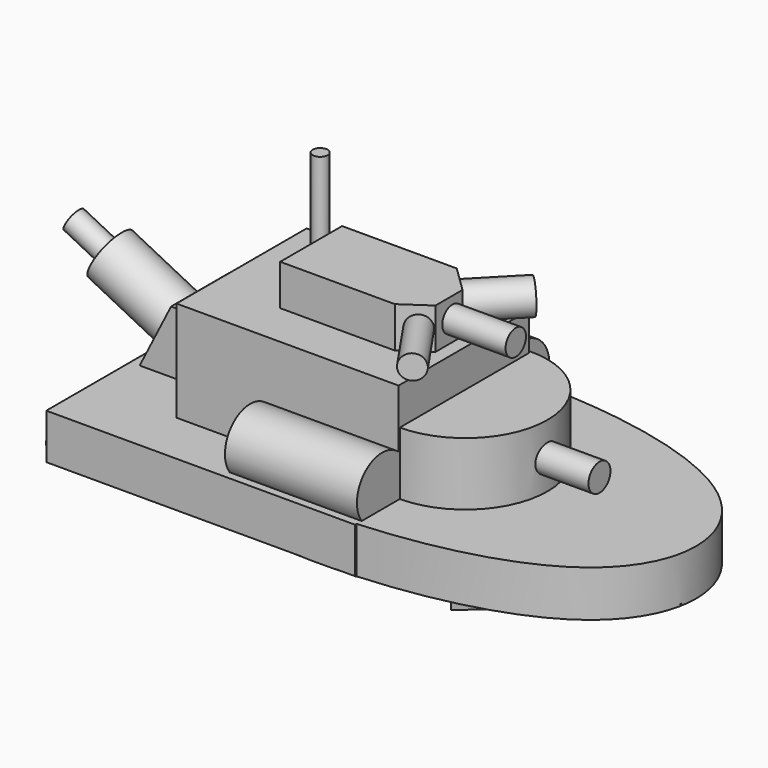
from build123d import *

# Parameters (mm, degrees)
F0_W      = 281.3238278031
F0_H      = 100.6183102727
F1_DEPTH  = 28.702
F3_DEPTH  = 192.024
F5_DEPTH  = 11.176
F6_DEPTH  = 16.51
F7_R      = 50.9790191052
F8_DEPTH  = 39.116
F9_W      = 138.0599290133
F9_H      = 101.1783219874
F10_DEPTH = 62.484
F11_R     = 8.5441952261
F12_DEPTH = 83.312
F13_W     = 61.6130270064
F13_H     = 25.6704241037
F14_DEPTH = 29.464
F15_W     = 38.1111055613
F15_H     = 22.8097289801
F16_DEPTH = 25.4
F17_R     = 21.1546629921
F18_DEPTH = 63.246
F19_R     = 19.5556802918
F20_DEPTH = 82.042
F21_W     = 71.2716747075
F21_H     = 48.0869095773
F22_DEPTH = 25.4
F23_R     = 7.9233421665
F24_DEPTH = 39.37
F25_R     = 7.5156557612
F26_DEPTH = 40.894
F27_R     = 10.3119477228
F28_DEPTH = 36.322
F29_W     = 44.719548896
F29_H     = 38.6362597346
F30_DEPTH = 28.702
F32_DEPTH = 44.958
F33_R     = 15.6273286388
F34_DEPTH = 49.53
F35_R     = 7.0493899226
F36_DEPTH = 25.4
F37_R     = 13.7507594289
F37_R_2   = 7.9743442037
F38_DEPTH = 37.592
F37_R_3   = 8.7506805575
F39_R     = 4.644151777
F40_DEPTH = 58.166


with BuildPart() as f1:
    # F0 (on Top) → F1 (new body)
    with BuildSketch(Plane.XY):
        with Locations((-24.3793539703, 0.1091174781)):
            Rectangle(F0_W, F0_H)
        with BuildLine():
            add(Edge.make_bspline(
                [(116.2825599313, 50.4182726145), (152.293026111, 22.4535704341), (152.293026111, -22.2353354778), (116.2825599313, -50.2000376582)],
                knots=[0.3128819291, 0.3128819291, 0.3128819291, 0.3128819291, 0.5, 0.5, 0.5, 0.5], degree=3))
            Line((116.2825599313, 50.4182726145), (116.2825599313, -50.2000376582))
        make_face()
        with BuildLine():
            Line((-165.0412678719, 50.4182726145), (116.2825599313, 50.4182726145))
            add(Edge.make_bspline(
                [(-165.0412678719, 50.4182726145), (-104.8278204483, 97.1783205419), (56.0691125078, 97.1783205419), (116.2825599313, 50.4182726145)],
                knots=[0, 0, 0, 0, 0.3128819291, 0.3128819291, 0.3128819291, 0.3128819291], degree=3))
        make_face()
        with BuildLine():
            Line((-165.0412678719, -50.2000376582), (-165.0412678719, 50.4182726145))
            add(Edge.make_bspline(
                [(-165.0412678719, -50.2000376582), (-201.0517340516, -22.2353354778), (-201.0517340516, 22.4535704341), (-165.0412678719, 50.4182726145)],
                knots=[0.8128819291, 0.8128819291, 0.8128819291, 0.8128819291, 1, 1, 1, 1], degree=3))
        make_face()
        with BuildLine():
            add(Edge.make_bspline(
                [(116.2825599313, -50.2000376582), (56.0691125078, -96.9600855856), (-104.8278204483, -96.9600855856), (-165.0412678719, -50.2000376582)],
                knots=[0.5, 0.5, 0.5, 0.5, 0.8128819291, 0.8128819291, 0.8128819291, 0.8128819291], degree=3))
            Line((116.2825599313, -50.2000376582), (-165.0412678719, -50.2000376582))
        make_face()
    extrude(amount=-F1_DEPTH)

    # F2 (on Right) → F3 (join)
    with BuildSketch(Plane.YZ):
        Polygon((84.8256722093, -28.180513531), (84.8256722093, 0), (-85.6735184789, 0), (-85.6735184789, -28.180513531), (0, -75.7616832852), align=None)
    extrude(amount=-F3_DEPTH)

    # F4 (on Front) → F5 (join)
    with BuildSketch(Plane.XZ):
        Polygon((0, -27.5897216052), (0, -77.0142525434), (142.4933820963, -27.5897216052), align=None)
    extrude(amount=F5_DEPTH)

    # F6 (add): a face of the model
    f6_faces = [f1.faces().sort_by_distance(p)[0] for p in [
        (46.4288760454, 0, -44.8060841811),
    ]]
    extrude(f6_faces, amount=F6_DEPTH)

    # F7 (on Top) → F8 (join)
    with BuildSketch(Plane.XY):
        Circle(F7_R)
    extrude(amount=F8_DEPTH)

    # F9 (on Top) → F10 (join)
    with BuildSketch(Plane.XY):
        with Locations((-69.0299645066, -1.3876985759)):
            Rectangle(F9_W, F9_H)
    extrude(amount=F10_DEPTH)

    # F11 (on Right) → F12 (join)
    with BuildSketch(Plane.YZ):
        with Locations((0, 18.2429812849)):
            Circle(F11_R)
    extrude(amount=F12_DEPTH)

    # F13 (on Top) → F14 (join)
    with BuildSketch(Plane.XY):
        with Locations((-44.9818205088, 61.9969516993)):
            Rectangle(F13_W, F13_H)
    extrude(amount=F14_DEPTH)

    # F15 (on Top) → F16 (join)
    with BuildSketch(Plane.XY):
        with Locations((-19.0555527806, -65.3974115849)):
            Rectangle(F15_W, F15_H)
    extrude(amount=F16_DEPTH)

    # F17 (on face) → F18 (join)
    with BuildSketch(Plane.YZ.offset(-14.1753070056)):
        with Locations((61.8273690343, 14.732)):
            Circle(F17_R)
    extrude(amount=-F18_DEPTH)

    # F19 (on face) → F20 (join)
    with BuildSketch(Plane.YZ):
        with Locations((-64.7612661123, 11.4093534648)):
            Circle(F19_R)
    extrude(amount=-F20_DEPTH)

    # F21 (on face) → F22 (join)
    with BuildSketch(Plane.XY.offset(62.484)):
        with Locations((-60.0350117311, -0.3072777763)):
            Rectangle(F21_W, F21_H)
        Polygon((-8.0839730799, 7.8503238037), (-24.3991743773, 23.7361770123), (-24.3991743773, -24.3507325649), (-8.0839730799, -13.1876999512), align=None)
    extrude(amount=F22_DEPTH)

    # F23 (on face) → F24 (join)
    with BuildSketch(Plane.YZ.offset(-8.0839730799)):
        with Locations((0, 75.184)):
            Circle(F23_R)
    extrude(amount=F24_DEPTH)

    # F25 (on face) → F26 (join)
    with BuildSketch(Plane(origin=(3.5682460915, -5.2151288342, 0), x_dir=(0.8253072578, 0.5646839207, 0), z_dir=(0.5646839207, -0.8253072578, 0))):
        with Locations((-22.2832337022, 75.184)):
            Circle(F25_R)
    extrude(amount=F26_DEPTH)

    # F27 (on face) → F28 (join)
    with BuildSketch(Plane(origin=(-0.0104526841, -0.0107351895, 0), x_dir=(-0.7164712032, 0.6976166677, 0), z_dir=(0.6976166677, 0.7164712032, 0))):
        with Locations((22.8173807263, 76.2572042043)):
            Circle(F27_R)
    extrude(amount=F28_DEPTH)

    # F29 (on face) → F30 (join)
    with BuildSketch(Plane(origin=(-138.0599290133, 0, 0), x_dir=(0, -1, 0), z_dir=(-1, 0, 0))):
        with Locations((-2.0744903013, 19.3181298673)):
            Rectangle(F29_W, F29_H)
    extrude(amount=F30_DEPTH)

    # F31 (on face) → F32 (join)
    with BuildSketch(Plane.XZ.offset(20.2852841467)):
        Polygon((-186.2631589174, 0), (-166.7619290133, 0), (-166.7619290133, 38.6362597346), align=None)
    extrude(amount=-F32_DEPTH)

    # F33 (on face) → F34 (join)
    with BuildSketch(Plane(origin=(-148.4450664661, 0, 74.9260251686), x_dir=(0, -1, 0), z_dir=(-0.8927285052, 0, 0.4505949577))):
        with Locations((0, -62.2898170892)):
            Circle(F33_R)
    extrude(amount=F34_DEPTH)

    # F35 (on face) → F36 (join)
    with BuildSketch(Plane(origin=(-192.6619093303, 0, 97.2439934257), x_dir=(0, -1, 0), z_dir=(-0.8927285052, 0, 0.4505949577))):
        with Locations((0, -62.2898170892)):
            Circle(F35_R)
    extrude(amount=F36_DEPTH)

    # F37 (on face) → F38 (join)
    with BuildSketch(Plane(origin=(-192.024, 0, 0), x_dir=(0, -1, 0), z_dir=(-1, 0, 0))):
        with Locations((0, -49.0443222225)):
            Circle(F37_R)
        with Locations((-31.330447644, -49.0443222225)):
            Circle(F37_R_2)
    extrude(amount=F38_DEPTH)

    # F39 (on face) → F40 (join)
    with BuildSketch(Plane.XY.offset(62.484)):
        with Locations((-112.9962727427, 28.3803287894)):
            Circle(F39_R)
    extrude(amount=F40_DEPTH)


with BuildPart() as f38:
    # F37 (on face) → F38, piece 2 (new body)
    with BuildSketch(Plane(origin=(-192.024, 0, 0), x_dir=(0, -1, 0), z_dir=(-1, 0, 0))):
        with Locations((30.0834812224, -49.0443222225)):
            Circle(F37_R_3)
    extrude(amount=F38_DEPTH)


solid = Compound([f1.part, f38.part])
